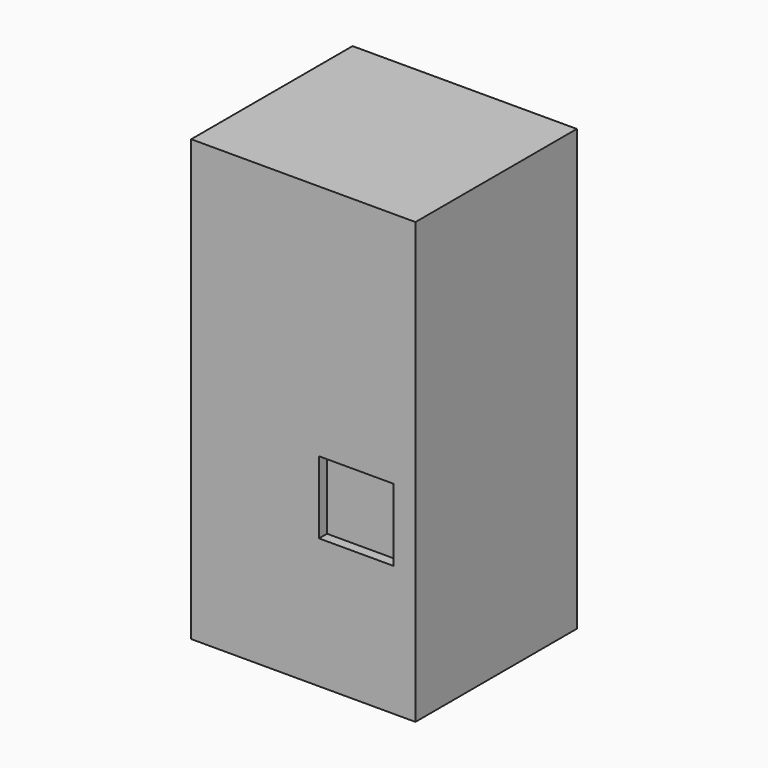
from build123d import *

# Parameters (mm, degrees)
F0_W     = 56.477651
F0_H     = 110.8297854662
F1_DEPTH = 50.8
F3_W     = 18.8258816488
F3_H     = 18.2185973972
F4_DEPTH = 2.54


with BuildPart() as f1:
    # F0 (on Front) → F1 (new body)
    with BuildSketch(Plane.XZ):
        Rectangle(F0_W, F0_H)
    extrude(amount=F1_DEPTH)

    # F3 (on face) → F4 (cut)
    with BuildSketch(Plane.XZ.offset(50.8)):
        with Locations((13.3603045251, -13.5121261701)):
            Rectangle(F3_W, F3_H)
    extrude(amount=-F4_DEPTH, mode=Mode.SUBTRACT)


solid = f1.part
